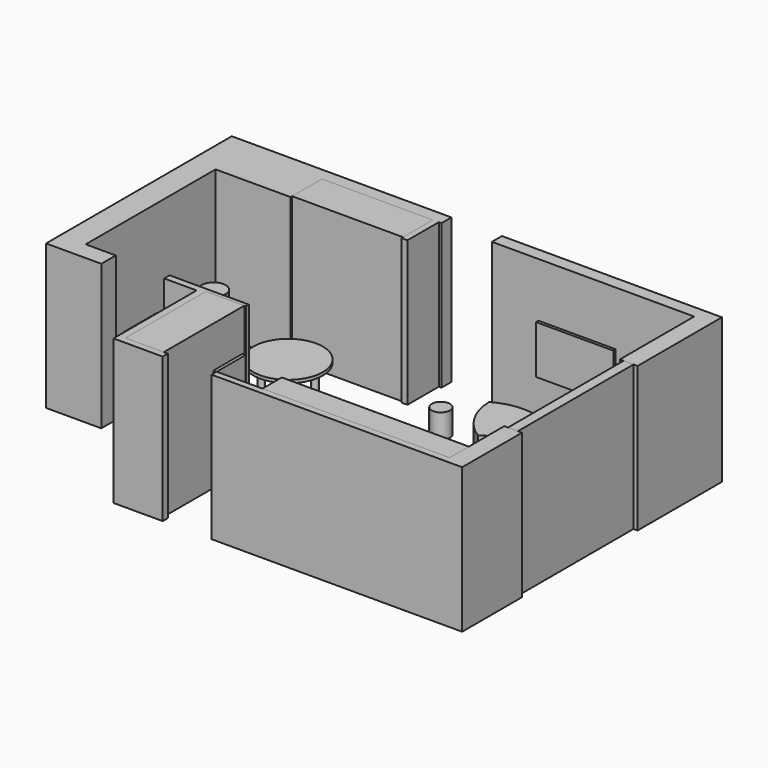
from build123d import *

# Parameters (mm, degrees)
F1_DEPTH  = 2400
F0_W      = 537.1888577938
F0_H      = 112.3662590981
F0_W_2    = 53.346157074
F0_H_2    = 600
F0_W_3    = 1250
F0_H_3    = 430
F0_W_4    = 550
F0_H_4    = 500
F2_DEPTH  = 900
F0_W_5    = 2000
F0_H_5    = 450
F0_R      = 50
F3_W      = 3100
F3_H      = 400
F4_DEPTH  = 800
F0_W_6    = 600
F0_H_6    = 650
F5_DEPTH  = 1900
F0_W_7    = 2100
F0_H_7    = 250
F6_DEPTH  = 900
F7_DEPTH  = 450
F0_W_8    = 350
F0_H_8    = 350
F8_DEPTH  = 910
F9_DEPTH  = 750
F10_DEPTH = 910
F11_W     = 450
F11_H     = 60
F12_DEPTH = 1000
F0_W_9    = 164.1221046448
F0_H_9    = 2394.7671353817
F13_DEPTH = 2400
F0_R_2    = 575
F14_DEPTH = 750
F15_DEPTH = 700
F0_W_10   = 1280
F0_H_10   = 50
F17_DEPTH = 1500
F18_W     = 1280
F18_H     = 700
F19_DEPTH = 50
F20_DEPTH = 400
F0_R_3    = 150
F0_H_11   = 400
F21_DEPTH = 1600
F22_W     = 580
F22_H     = 540
F22_H_2   = 500
F23_DEPTH = 380
F24_W     = 600
F24_H     = 600
F25_DEPTH = 25
F24_W_2   = 3100
F24_H_2   = 100
F26_DEPTH = 30
F27_W     = 10
F27_H     = 800
F28_DEPTH = 10
F29_W     = 700
F29_H     = 600
F30_DEPTH = 60
F0_W_11   = 1835.4965090752
F0_H_12   = 616.584777832
F31_DEPTH = 2400
F0_R_4    = 200
F32_DEPTH = 1000


# Not quite as in the source:
# - a feature names something its author has since deleted; it is built from what else it names


with BuildPart() as f1:
    # F0 (on Top) → F1 (new body)
    with BuildSketch(Plane.XY):
        Polygon((5332.8738090396, 2704.7533988953), (5394.4396972656, 2704.7533988952), (5558.5618019104, 2704.7533988953), (5626.5387535095, 2704.7533988953), (5626.5387535095, 4450.9944915771), (5332.8738090396, 4450.9944915771), (5332.8738090396, 4243.6318397522), align=None)
        Polygon((4032.8738090396, 4243.6318397522), (5332.8738090396, 4243.6318397522), (5332.8738090396, 4450.9944915771), (1981.1851978302, 4450.9944915771), (1981.1851978302, 4243.6318397522), (2752.8738090396, 4243.6318397522), align=None)
    extrude(amount=F1_DEPTH)


with BuildPart() as f1b:
    # F0 (on Top) → F1, piece 2 (new body)
    with BuildSketch(Plane.XY):
        Polygon((5332.8738090396, -222.1663832664), (5332.8738090396, -822.1663832664), (2232.8738090396, -822.1663832664), (1474.7484922409, -822.1663832664), (1474.7484922409, -928.7706017494), (5626.5387535095, -928.7706017494), (5626.5387535095, 309.9862635136), (5558.5618019104, 309.9862635135), (5394.4396972656, 309.9862635135), (5332.8738090396, 309.9862635136), align=None)
    extrude(amount=F1_DEPTH)


with BuildPart() as f1c:
    # F0 (on Top) → F1, piece 3 (new body)
    with BuildSketch(Plane.XY):
        Polygon((597.9725122452, -822.1663832664), (-37.1261909604, -822.1663832664), (-37.1261909604, -26.347534731), (-37.1261909604, 845.5312275887), (-37.1261909604, 905.5312275887), (-150.5666673183, 905.5312275887), (-150.5666673183, 793.1649684906), (-150.5666673183, -928.7706017494), (664.8011207581, -928.7706017494), (664.8011207581, -822.1663832664), align=None)
        with Locations((-419.1610962152, 849.3480980396)):
            Rectangle(F0_W, F0_H)
        Polygon((-37.1261909604, 845.5312275887), (597.9725122452, 845.5312275887), (624.0934729576, 845.5312275887), (624.0934729576, 905.5312275887), (597.9725122452, 905.5312275887), (-37.1261909604, 905.5312275887), align=None)
    extrude(amount=F1_DEPTH)


with BuildPart() as f1d:
    # F0 (on Top) → F1, piece 4 (new body)
    with BuildSketch(Plane.XY):
        with Locations((1448.0754137039, -522.1663832664)):
            Rectangle(F0_W_2, F0_H_2)
    extrude(amount=F1_DEPTH)


with BuildPart() as f1e:
    # F0 (on Top) → F1, piece 5 (new body)
    with BuildSketch(Plane.XY):
        Polygon((1101.2586355209, 4243.6318397522), (1145.4427242279, 4243.6318397522), (1145.4427242279, 4450.9944915771), (-2494.3199157715, 4450.9944915771), (-2494.3199157715, 605.3053736687), (-1579.2272090912, 605.3053736687), (-1579.2272090912, 905.5312275887), (-2078.3698558807, 905.5312275887), (-2078.3698558807, 3594.8448181152), (-834.2378735542, 3594.8448181152), (-834.2378735542, 3627.0470619202), (-834.2378735542, 4243.6318397522), (1001.2586355209, 4243.6318397522), align=None)
        Polygon((1101.2586355209, 3594.8448181152), (1101.2586355209, 4243.6318397522), (1001.2586355209, 4243.6318397522), (1001.2586355209, 3627.0470619202), (1001.2586355209, 3594.8448181152), align=None)
    extrude(amount=F1_DEPTH)


with BuildPart() as f2:
    # F0 (on Top) → F2 (new body)
    with BuildSketch(Plane.XY):
        Polygon((2232.8738090396, -822.1663832664), (5332.8738090396, -822.1663832664), (5332.8738090396, -222.1663832664), (4732.8738090396, -222.1663832664), (2232.8738090396, -222.1663832664), align=None)
        with Locations((2957.8738090396, -517.1663832664)):
            Rectangle(F0_W_3, F0_H_3, mode=Mode.SUBTRACT)
        with Locations((4757.8738090396, -522.1663832664)):
            Rectangle(F0_W_4, F0_H_4, mode=Mode.SUBTRACT)
    extrude(amount=F2_DEPTH)

    # F0 (on Top) → F8 (join)
    with BuildSketch(Plane.XY):
        with Locations((2957.8738090396, -517.1663832664)):
            Rectangle(F0_W_3, F0_H_3)
        with Locations((2957.8738090396, -507.1663832664)):
            Rectangle(F0_W_8, F0_H_8, mode=Mode.SUBTRACT)
        with Locations((3357.8738090396, -507.1663832664)):
            Rectangle(F0_W_8, F0_H_8, mode=Mode.SUBTRACT)
    extrude(amount=F8_DEPTH)

    # F0 (on Top) → F9 (join)
    with BuildSketch(Plane.XY):
        with Locations((3357.8738090396, -507.1663832664)):
            Rectangle(F0_W_8, F0_H_8)
        with Locations((2957.8738090396, -507.1663832664)):
            Rectangle(F0_W_8, F0_H_8)
    extrude(amount=F9_DEPTH)

    # F0 (on Top) → F10 (join)
    with BuildSketch(Plane.XY):
        with Locations((4757.8738090396, -522.1663832664)):
            Rectangle(F0_W_4, F0_H_4)
    extrude(amount=F10_DEPTH)

    # F24 (on face) → F25 (join)
    with BuildSketch(Plane(origin=(0, -222.1663832664, 0), x_dir=(-1, 0, 0), z_dir=(0, 1, 0))):
        with Locations((-4832.8738090396, 500)):
            Rectangle(F24_W, F24_H)
        with Locations((-4032.8738090396, 500)):
            Rectangle(F24_W, F24_H)
    extrude(amount=F25_DEPTH)

    # F24 (on face) → F26 (cut)
    with BuildSketch(Plane(origin=(0, -222.1663832664, 0), x_dir=(-1, 0, 0), z_dir=(0, 1, 0))):
        with Locations((-3782.8738090396, 50)):
            Rectangle(F24_W_2, F24_H_2)
    extrude(amount=-F26_DEPTH, mode=Mode.SUBTRACT)


with BuildPart() as f2b:
    # F0 (on Top) → F2, piece 2 (new body)
    with BuildSketch(Plane.XY):
        with Locations((3647.4789381027, 902.8336167336)):
            Rectangle(F0_W_5, F0_H_5)
    extrude(amount=F2_DEPTH)


with BuildPart() as f2c:
    # F0 (on Top) → F2, piece 3 (new body)
    with BuildSketch(Plane.XY):
        with Locations((1847.4789381027, 902.8336167336)):
            Circle(F0_R)
    extrude(amount=F2_DEPTH)


with BuildPart() as f4:
    # F3 (on face) → F4 (new body)
    with BuildSketch(Plane.XY.offset(2400)):
        with Locations((3782.8738090396, -622.1663832664)):
            Rectangle(F3_W, F3_H)
    extrude(amount=-F4_DEPTH)

    # F27 (on face) → F28 (cut)
    with BuildSketch(Plane(origin=(0, -422.1663832664, 0), x_dir=(-1, 0, 0), z_dir=(0, 1, 0))):
        with Locations((-2737.8738090396, 2000)):
            Rectangle(F27_W, F27_H)
        with Locations((-3247.8738090396, 2000)):
            Rectangle(F27_W, F27_H)
        with Locations((-3757.8738090396, 2000)):
            Rectangle(F27_W, F27_H)
        with Locations((-4267.8738090396, 2000)):
            Rectangle(F27_W, F27_H)
        with Locations((-4777.8738090396, 2000)):
            Rectangle(F27_W, F27_H)
    extrude(amount=-F28_DEPTH, mode=Mode.SUBTRACT)


with BuildPart() as f5:
    # F0 (on Top) → F5 (new body)
    with BuildSketch(Plane.XY):
        with Locations((1811.9415521622, -467.1663832664)):
            Rectangle(F0_W_6, F0_H_6)
    extrude(amount=F5_DEPTH)


with BuildPart() as f6:
    # F0 (on Top) → F6 (new body)
    with BuildSketch(Plane.XY):
        with Locations((3682.8738090396, 1352.8336167336)):
            Rectangle(F0_W_7, F0_H_7)
    extrude(amount=F6_DEPTH)

    # F0 (on Top) → F7 (join)
    with BuildSketch(Plane.XY):
        Polygon((2632.8738090396, 1477.8336167336), (4732.8738090396, 1477.8336167336), (4732.8738090396, 2727.8336167336), (3932.8738090396, 2727.8336167336), (3932.8738090396, 2087.8336167336), (2632.8738090396, 2087.8336167336), align=None)
    extrude(amount=F7_DEPTH)


with BuildPart() as f12:
    # F11 (on face) → F12 (new body)
    with BuildSketch(Plane(origin=(2647.4789381027, 0, 0), x_dir=(0, -1, 0), z_dir=(-1, 0, 0))):
        with Locations((-902.8336167336, 870)):
            Rectangle(F11_W, F11_H)
    extrude(amount=F12_DEPTH)


with BuildPart() as f13:
    # F0 (on Top) → F13 (new body)
    with BuildSketch(Plane.XY):
        with Locations((5476.500749588, 1507.3698312044)):
            Rectangle(F0_W_9, F0_H_9)
    extrude(amount=F13_DEPTH)


with BuildPart() as f14:
    # F0 (on Top) → F14 (new body)
    with BuildSketch(Plane.XY):
        with Locations((0, 2500.5469322205)):
            Circle(F0_R_2)
        with Locations((-247.4873734153, 2253.0595588052)):
            Circle(F0_R, mode=Mode.SUBTRACT)
        with Locations((247.4873734153, 2253.0595588052)):
            Circle(F0_R, mode=Mode.SUBTRACT)
        with Locations((-247.4873734153, 2748.0343056358)):
            Circle(F0_R, mode=Mode.SUBTRACT)
        with Locations((247.4873734153, 2748.0343056358)):
            Circle(F0_R, mode=Mode.SUBTRACT)
        with Locations((247.4873734153, 2748.0343056358)):
            Circle(F0_R)
        with Locations((247.4873734153, 2253.0595588052)):
            Circle(F0_R)
        with Locations((-247.4873734153, 2748.0343056358)):
            Circle(F0_R)
        with Locations((-247.4873734153, 2253.0595588052)):
            Circle(F0_R)
    extrude(amount=F14_DEPTH)


with BuildPart() as f15:
    # F0 (on Top) → F15 (new body)
    with BuildSketch(Plane.XY):
        with Locations((0, 2500.5469322205)):
            Circle(F0_R_2)
        with Locations((-247.4873734153, 2253.0595588052)):
            Circle(F0_R, mode=Mode.SUBTRACT)
        with Locations((247.4873734153, 2253.0595588052)):
            Circle(F0_R, mode=Mode.SUBTRACT)
        with Locations((-247.4873734153, 2748.0343056358)):
            Circle(F0_R, mode=Mode.SUBTRACT)
        with Locations((247.4873734153, 2748.0343056358)):
            Circle(F0_R, mode=Mode.SUBTRACT)
    extrude(amount=F15_DEPTH)


with BuildPart() as f14_1:
    add(f14.part)

    # F16: cut F15
    add(f15.part, mode=Mode.SUBTRACT)


with BuildPart() as f17:
    # F0 (on Top) → F17 (new body)
    with BuildSketch(Plane.XY):
        with Locations((3392.8738090396, 4218.6318397522)):
            Rectangle(F0_W_10, F0_H_10)
    extrude(amount=F17_DEPTH)

    # F18 (on face) → F19 (cut)
    with BuildSketch(Plane.XZ.offset(-4193.6318397522)):
        with Locations((3392.8738090396, 350)):
            Rectangle(F18_W, F18_H)
    extrude(amount=-F19_DEPTH, mode=Mode.SUBTRACT)


with BuildPart() as f20:
    # F0 (on Top) → F20 (new body)
    with BuildSketch(Plane.XY):
        with BuildLine():
            ThreePointArc((2356.5598369582, 3718.6318397522), (2490.1661397403, 3245.7694746289), (2832.8738090396, 2893.6318397522))
            ThreePointArc((2832.8738090396, 2893.6318397522), (3175.5814783389, 3245.7694746289), (3309.187781121, 3718.6318397522))
            ThreePointArc((3309.187781121, 3718.6318397522), (2832.8738090396, 3839.3565699987), (2356.5598369582, 3718.6318397522))
        make_face()
    extrude(amount=F20_DEPTH)


with BuildPart() as f20b:
    # F0 (on Top) → F20, piece 2 (new body)
    with BuildSketch(Plane.XY):
        with Locations((4030.5371284485, 3705.1014900208)):
            Circle(F0_R_3)
    extrude(amount=F20_DEPTH)


with BuildPart() as f20c:
    # F0 (on Top) → F20, piece 3 (new body)
    with BuildSketch(Plane.XY):
        with Locations((1959.0933322906, 3213.9573097229)):
            Circle(F0_R_3)
    extrude(amount=F20_DEPTH)


with BuildPart() as f21:
    # F0 (on Top) → F21 (new body)
    with BuildSketch(Plane.XY):
        with Locations((5001.082611084, 4008.5523605347)):
            Rectangle(F0_W_6, F0_H_11)
    extrude(amount=F21_DEPTH)

    # F22 (on face) → F23 (cut)
    with BuildSketch(Plane.XZ.offset(-3808.5523605347)):
        with Locations((5001.082611084, 1320)):
            Rectangle(F22_W, F22_H)
        with Locations((5001.082611084, 780)):
            Rectangle(F22_W, F22_H_2)
        with Locations((5001.082611084, 260)):
            Rectangle(F22_W, F22_H_2)
    extrude(amount=-F23_DEPTH, mode=Mode.SUBTRACT)


with BuildPart() as f30:
    # F29 (on face) → F30 (new body)
    with BuildSketch(Plane.YZ.offset(-2078.3698558807)):
        with Locations((2026.7077445984, 500)):
            Rectangle(F29_W, F29_H)
    extrude(amount=F30_DEPTH)


with BuildPart() as f31:
    # F0 (on Top) → F31 (new body)
    with BuildSketch(Plane.XY):
        with Locations((83.5103809834, 3935.3394508362)):
            Rectangle(F0_W_11, F0_H_12)
    extrude(amount=F31_DEPTH)


with BuildPart() as f31b:
    # F0 (on Top) → F31, piece 2 (new body)
    with BuildSketch(Plane.XY):
        Polygon((-37.1261909604, -26.347534731), (-37.1261909604, -822.1663832664), (597.9725122452, -822.1663832664), (597.9725122452, 845.5312275887), (-37.1261909604, 845.5312275887), align=None)
    extrude(amount=F31_DEPTH)


with BuildPart() as f32:
    # F0 (on Top) → F32 (new body)
    with BuildSketch(Plane.XY):
        with Locations((-1673.9757061005, 3049.9031543732)):
            Circle(F0_R_4)
    extrude(amount=F32_DEPTH)


solid = Compound([f1.part, f1b.part, f1c.part, f1d.part, f1e.part, f2.part, f2b.part, f2c.part, f4.part, f5.part, f6.part, f12.part, f13.part, f14_1.part, f17.part, f20.part, f20b.part, f20c.part, f21.part, f30.part, f31.part, f31b.part, f32.part])
